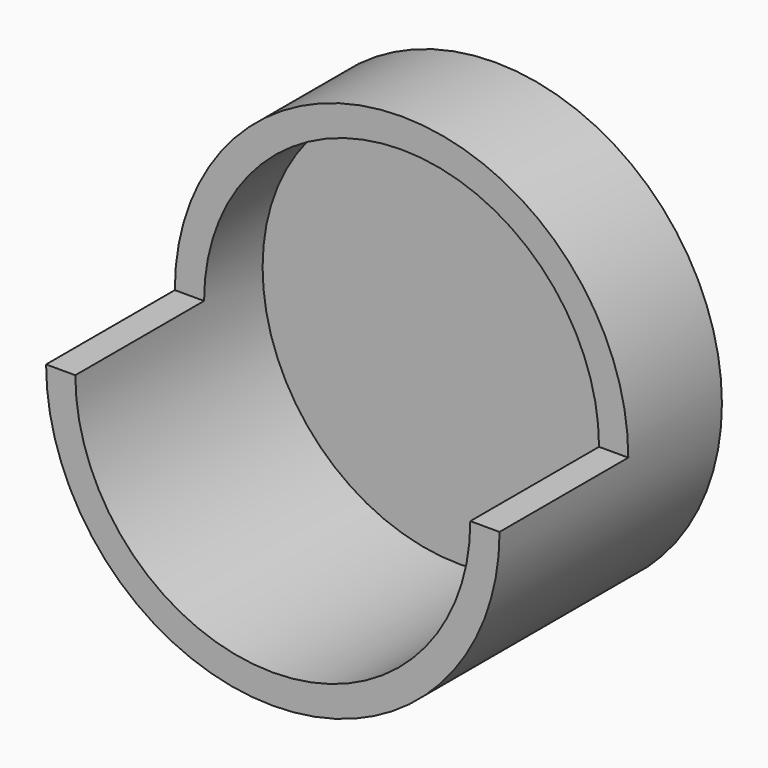
from build123d import *

# Parameters (mm, degrees)
F1_DEPTH = 16
F2_DEPTH = 3
F4_DEPTH = 8


with BuildPart() as f1:
    # F0 (on Front) → F1 (new body)
    with BuildSketch(Plane.XZ):
        with BuildLine():
            Line((15.5, 0), (13.5, 0))
            ThreePointArc((13.5, 0), (0, -13.5), (-13.5, 0))
            Line((-13.5, 0), (-15.5, 0))
            ThreePointArc((-15.5, 0), (0, -15.5), (15.5, 0))
        make_face()
    extrude(amount=F1_DEPTH)

    # F0 (on Front) → F2 (join)
    with BuildSketch(Plane.XZ):
        with BuildLine():
            Line((15.5, 0), (13.5, 0))
            ThreePointArc((13.5, 0), (0, -13.5), (-13.5, 0))
            Line((-13.5, 0), (-15.5, 0))
            ThreePointArc((-15.5, 0), (0, -15.5), (15.5, 0))
        make_face()
        with BuildLine():
            ThreePointArc((-13.5, 0), (0, -13.5), (13.5, 0))
            ThreePointArc((13.5, 0), (0, 13.5), (-13.5, 0))
        make_face()
    extrude(amount=-F2_DEPTH)

    # F3 (on face) → F4 (join)
    with BuildSketch(Plane(origin=(0, 3, 0), x_dir=(-1, 0, 0), z_dir=(0, 1, 0))):
        with BuildLine():
            Line((13.5, 0), (15.5, 0))
            ThreePointArc((15.5, 0), (0, 15.5), (-15.5, 0))
            Line((-15.5, 0), (-13.5, 0))
            ThreePointArc((-13.5, 0), (0, 13.5), (13.5, 0))
        make_face()
    extrude(amount=-F4_DEPTH)


solid = f1.part
